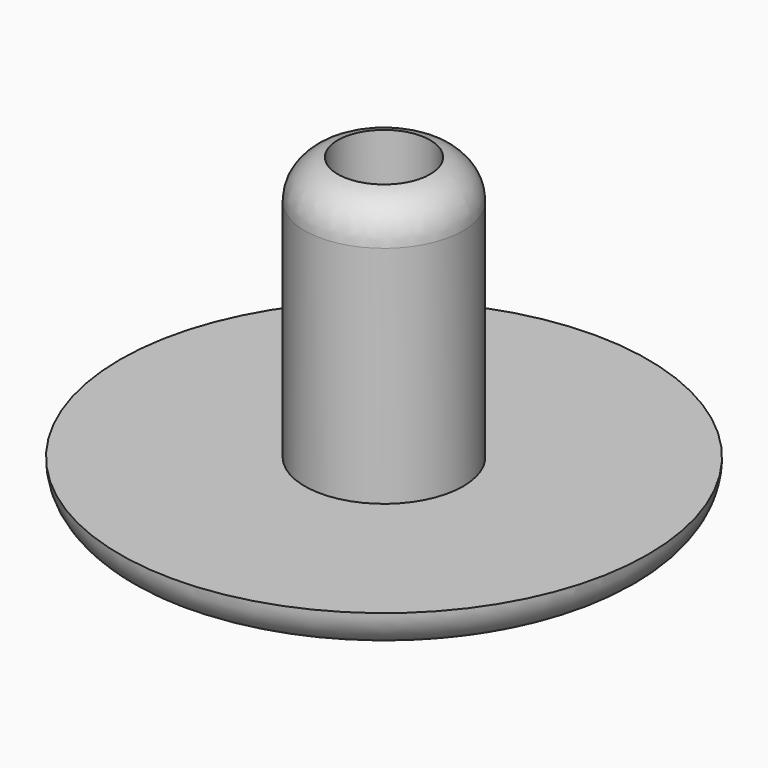
from build123d import *

# Parameters (mm, degrees)
F0_R     = 10
F1_DEPTH = 1.5
F2_R     = 3
F3_DEPTH = 10
F4_R     = 1.75
F5_DEPTH = 11.501


# Not quite as in the source:
# - a fillet or chamfer that OpenCascade refuses, or shapes differently, is made with other operations: its cross-section is extruded or revolved along the edge and cut away or added


with BuildPart() as f1:
    # F0 (on Top) → F1 (new body)
    with BuildSketch(Plane.XY):
        Circle(F0_R)
    extrude(amount=F1_DEPTH)

    # F2 (on face) → F3 (join)
    with BuildSketch(Plane.XY.offset(1.5)):
        Circle(F2_R)
    extrude(amount=F3_DEPTH)

    # F4 (on face) → F5 (cut, through all)
    with BuildSketch(Plane.XY.offset(11.5)):
        Circle(F4_R)
    extrude(amount=-F5_DEPTH, mode=Mode.SUBTRACT)

    # F6: fillet of radius 1.5 on 3 edges, made by hand

    # F6_s1 → F6_t2 (revolve, cut)
    with BuildSketch(Plane.XZ):
        with BuildLine():
            ThreePointArc((10, 1.5), (9.5606601718, 0.4393398282), (8.5, 0))
            Line((8.5, 0), (10, 0))
            Line((10, 0), (10, 1.5))
        make_face()
    revolve(axis=Axis((0, 0, 0), (0, 0, 1)), mode=Mode.SUBTRACT)

    # F6_s3 → F6_t4 (revolve, cut)
    with BuildSketch(Plane.XZ):
        with BuildLine():
            ThreePointArc((3.25, 0), (2.1893398282, 0.4393398282), (1.75, 1.5))
            Line((1.75, 1.5), (1.75, 0))
            Line((1.75, 0), (3.25, 0))
        make_face()
    revolve(axis=Axis((0, 0, 0), (0, 0, 1)), mode=Mode.SUBTRACT)

    # F6_s5 → F6_t6 (revolve, cut)
    with BuildSketch(Plane.XZ):
        with BuildLine():
            ThreePointArc((3, 10.0209800542), (2.6456439237, 10.9892258908), (1.75, 11.5))
            Line((1.75, 11.5), (3, 11.5))
            Line((3, 11.5), (3, 10.0209800542))
        make_face()
    revolve(axis=Axis((0, 0, 11.5), (0, 0, 1)), mode=Mode.SUBTRACT)


solid = f1.part
